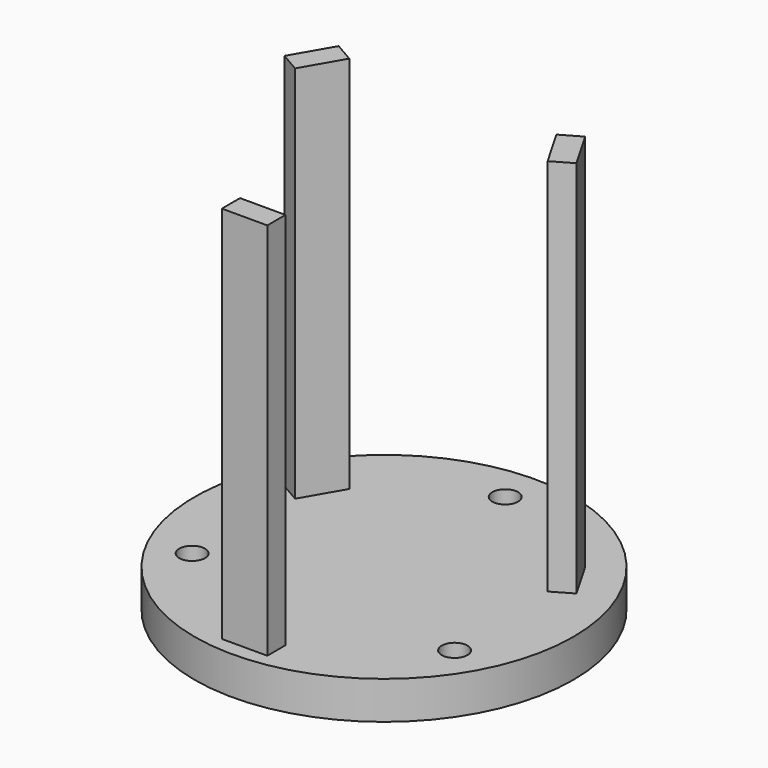
from build123d import *

# Parameters (mm, degrees)
F0_R     = 25
F0_R_2   = 1.7
F1_DEPTH = 5
F3_W     = 6
F3_H     = 3
F4_DEPTH = 50


# Not quite as in the source:
# - a feature names something its author has since deleted; it is built from what else it names


with BuildPart() as f1:
    # F0 (on Top) → F1 (new body)
    with BuildSketch(Plane.XY):
        Circle(F0_R)
        with Locations((-17.3205080757, -10)):
            Circle(F0_R_2, mode=Mode.SUBTRACT)
        with Locations((17.3205080757, -10)):
            Circle(F0_R_2, mode=Mode.SUBTRACT)
        with Locations((0, 20)):
            Circle(F0_R_2, mode=Mode.SUBTRACT)
    extrude(amount=F1_DEPTH)

    # F3 (on face) → F4 (join)
    with BuildSketch(Plane.XY.offset(5)):
        Polygon((-16.6554445662, 6.1519237886), (-13.6554445662, 11.3480762114), (-16.2535207776, 12.8480762114), (-19.2535207776, 7.6519237886), align=None)
        Polygon((16.2017059222, 12.9378221735), (13.6036297108, 11.4378221735), (16.6036297108, 6.2416697508), (19.2017059222, 7.7416697508), align=None)
        with Locations((0, -21.5)):
            Rectangle(F3_W, F3_H)
    extrude(amount=F4_DEPTH)


solid = f1.part
